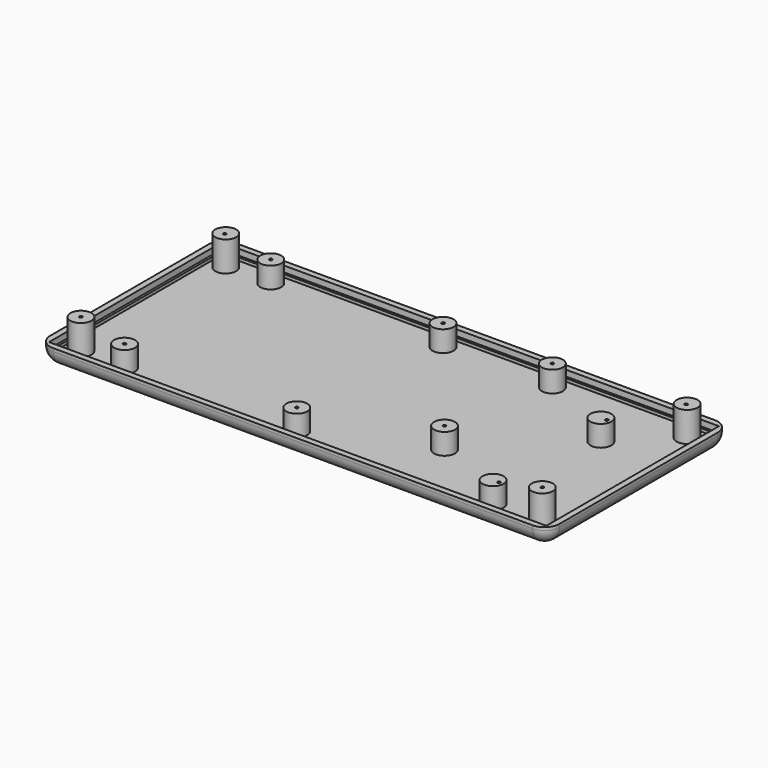
from build123d import *

# Parameters (mm, degrees)
F0_W            = 170
F0_H            = 76
F1_DEPTH        = 6
F2_W            = 164.4
F2_H            = 70.4
F3_DEPTH        = 3
F4_R            = 3.5
F5_DEPTH        = 7
F6_R            = 4
F7_DEPTH        = 2.8
F8_W            = 166
F8_H            = 72
F8_W_2          = 163.2
F8_H_2          = 69.2
F9_DEPTH        = 2
F10_R           = 3.5
F11_DEPTH       = 10
F12_R           = 0.5
F13_DEPTH       = 0.5
F14_R           = 0.5
F15_DEPTH       = 0.5
F17_D           = 3
F17_DEPTH       = 2.5
F17_CSINK_D     = 6.72
F17_CSINK_ANGLE = 90
F17_TIP         = 0.9012909285
F18_T1_DEPTH    = 13.5
F18_T3_DEPTH    = 66
F18_T5_DEPTH    = 160
F18_S9_W        = 5
F18_S9_H        = 5
F18_T10_DEPTH   = 5
F18_S15_W       = 5
F18_S15_H       = 5
F18_T16_DEPTH   = 5
F18_S21_W       = 5
F18_S21_H       = 5
F18_T22_DEPTH   = 5
F18_S27_W       = 5
F18_S27_H       = 5
F18_T28_DEPTH   = 5


# Not quite as in the source:
# - a fillet or chamfer that OpenCascade refuses, or shapes differently, is made with other operations: its cross-section is extruded or revolved along the edge and cut away or added


with BuildPart() as f1:
    # F0 (on Top) → F1 (new body)
    with BuildSketch(Plane.XY):
        with Locations((85, 38)):
            Rectangle(F0_W, F0_H)
    extrude(amount=F1_DEPTH)

    # F2 (on face) → F3 (cut)
    with BuildSketch(Plane.XY.offset(6)):
        with Locations((85, 38)):
            Rectangle(F2_W, F2_H)
    extrude(amount=-F3_DEPTH, mode=Mode.SUBTRACT)

    # F4 (on face) → F5 (join)
    with BuildSketch(Plane.XY.offset(3)):
        with Locations((22.8, 68.5)):
            Circle(F4_R)
        with Locations((22.8, 7.5)):
            Circle(F4_R)
        with Locations((80.3, 68.5)):
            Circle(F4_R)
        with Locations((80.3, 7.5)):
            Circle(F4_R)
        with Locations((116.8, 68.5)):
            Circle(F4_R)
        with Locations((145.8, 52.5)):
            Circle(F4_R)
        with Locations((116.8, 23.5)):
            Circle(F4_R)
        with Locations((145.8, 7.5)):
            Circle(F4_R)
    extrude(amount=F5_DEPTH)

    # F6 (on face) → F7 (cut, through all)
    with BuildSketch(Plane(origin=(0, 0, 0), x_dir=(0, -1, 0), z_dir=(-1, 0, 0))):
        with Locations((-57, 18)):
            Circle(F6_R)
        with Locations((-19, 18)):
            Circle(F6_R)
    extrude(amount=-F7_DEPTH, mode=Mode.SUBTRACT)

    # F8 (on face) → F9 (cut)
    with BuildSketch(Plane.XY.offset(6)):
        with Locations((85, 38)):
            Rectangle(F8_W, F8_H)
        with Locations((84.6, 37.6)):
            Rectangle(F8_W_2, F8_H_2, mode=Mode.SUBTRACT)
    extrude(amount=-F9_DEPTH, mode=Mode.SUBTRACT)

    # F10 (on face) → F11 (join)
    with BuildSketch(Plane.XY.offset(3)):
        with Locations((8, 68.2)):
            Circle(F10_R)
        with Locations((8, 7.8)):
            Circle(F10_R)
        with Locations((162, 7.8)):
            Circle(F10_R)
        with Locations((162, 68.2)):
            Circle(F10_R)
    extrude(amount=F11_DEPTH)

    # F12 (on face) → F13 (cut)
    with BuildSketch(Plane.XY.offset(13)):
        with Locations((8, 67.8)):
            Circle(F12_R)
        with Locations((8, 7.8)):
            Circle(F12_R)
        with Locations((162, 7.8)):
            Circle(F12_R)
        with Locations((162, 67.8)):
            Circle(F12_R)
    extrude(amount=-F13_DEPTH, mode=Mode.SUBTRACT)

    # F14 (on face) → F15 (cut)
    with BuildSketch(Plane.XY.offset(10)):
        with Locations((22.8, 68.5)):
            Circle(F14_R)
        with Locations((22.8, 7.5)):
            Circle(F14_R)
        with Locations((80.3, 68.5)):
            Circle(F14_R)
        with Locations((80.3, 7.5)):
            Circle(F14_R)
        with Locations((116.8, 68.5)):
            Circle(F14_R)
        with Locations((147.8, 52.5)):
            Circle(F14_R)
        with Locations((116.8, 23.5)):
            Circle(F14_R)
        with Locations((147.8, 7.5)):
            Circle(F14_R)
    extrude(amount=-F15_DEPTH, mode=Mode.SUBTRACT)

    # F17
    with Locations(Plane(origin=(0, 0, 0), x_dir=(1, 0, 0), z_dir=(0, 0, -1))):
        with Locations((8, -8), (8, -68), (162, -68), (162, -8)):
            CounterSinkHole(F17_D / 2, F17_CSINK_D / 2, depth=F17_DEPTH, counter_sink_angle=F17_CSINK_ANGLE)
            with Locations((0, 0, -(F17_DEPTH + F17_TIP / 2))):  # 118° drill point
                Cone(0, F17_D / 2, F17_TIP, mode=Mode.SUBTRACT)

    # F18: fillet of radius 5 on 8 edges, made by hand

    # F18_s2 → F18_t1 (cut)
    with BuildSketch(Plane.XY.offset(5)):
        with BuildLine():
            ThreePointArc((165, 76), (168.5355339059, 74.5355339059), (170, 71))
            Line((170, 71), (170, 76))
            Line((170, 76), (165, 76))
        make_face()
        with BuildLine():
            ThreePointArc((165, 0), (168.5355339059, 1.4644660941), (170, 5))
            Line((170, 5), (170, 0))
            Line((170, 0), (165, 0))
        make_face()
        with BuildLine():
            ThreePointArc((0, 71), (1.4644660941, 74.5355339059), (5, 76))
            Line((5, 76), (0, 76))
            Line((0, 76), (0, 71))
        make_face()
        with BuildLine():
            ThreePointArc((0, 5), (1.4644660941, 1.4644660941), (5, 0))
            Line((5, 0), (0, 0))
            Line((0, 0), (0, 5))
        make_face()
    extrude(amount=F18_T1_DEPTH, mode=Mode.SUBTRACT)

    # F18_s4 → F18_t3 (cut)
    with BuildSketch(Plane.XZ.offset(-71)):
        with BuildLine():
            ThreePointArc((165, 0), (168.5355339059, 1.4644660941), (170, 5))
            Line((170, 5), (170, 0))
            Line((170, 0), (165, 0))
        make_face()
        with BuildLine():
            ThreePointArc((0, 5), (1.4644660941, 1.4644660941), (5, 0))
            Line((5, 0), (0, 0))
            Line((0, 0), (0, 5))
        make_face()
    extrude(amount=F18_T3_DEPTH, mode=Mode.SUBTRACT)

    # F18_s6 → F18_t5 (cut)
    with BuildSketch(Plane.YZ.offset(5)):
        with BuildLine():
            ThreePointArc((76, 5), (74.5355339059, 1.4644660941), (71, 0))
            Line((71, 0), (76, 0))
            Line((76, 0), (76, 5))
        make_face()
        with BuildLine():
            ThreePointArc((0, 5), (1.4644660941, 1.4644660941), (5, 0))
            Line((5, 0), (0, 0))
            Line((0, 0), (0, 5))
        make_face()
    extrude(amount=F18_T5_DEPTH, mode=Mode.SUBTRACT)


with BuildPart() as f18_tool8:
    # F18_s9 → F18_t10 (new body)
    with BuildSketch(Plane.XZ.offset(-71)):
        with Locations((167.5, 2.5)):
            Rectangle(F18_S9_W, F18_S9_H)
    extrude(amount=-F18_T10_DEPTH)

    # F18_s11 → F18_t12 (revolve, cut)
    with BuildSketch(Plane(origin=(165, 71, 5), x_dir=(-0.7071067812, 0, 0.7071067812), z_dir=(-0.7071067812, 0, -0.7071067812))):
        with BuildLine():
            ThreePointArc((0, -5), (5, 0), (0, 5))
            Line((0, 5), (0, -5))
        make_face()
    revolve(axis=Axis((165, 71, 5), (0, 1, 0)), mode=Mode.SUBTRACT)


with BuildPart() as f1_1:
    add(f1.part)

    # F18_t7: cut F18_tool8
    add(f18_tool8.part, mode=Mode.SUBTRACT)


with BuildPart() as f18_tool14:
    # F18_s15 → F18_t16 (new body)
    with BuildSketch(Plane.XZ.offset(-5)):
        with Locations((167.5, 2.5)):
            Rectangle(F18_S15_W, F18_S15_H)
    extrude(amount=F18_T16_DEPTH)

    # F18_s17 → F18_t18 (revolve, cut)
    with BuildSketch(Plane(origin=(165, 5, 5), x_dir=(-0.7071067812, 0, 0.7071067812), z_dir=(0.7071067812, 0, 0.7071067812))):
        with BuildLine():
            ThreePointArc((0, -5), (5, 0), (0, 5))
            Line((0, 5), (0, -5))
        make_face()
    revolve(axis=Axis((165, 5, 5), (0, -1, 0)), mode=Mode.SUBTRACT)


with BuildPart() as f1_2:
    add(f1_1.part)

    # F18_t13: cut F18_tool14
    add(f18_tool14.part, mode=Mode.SUBTRACT)


with BuildPart() as f18_tool20:
    # F18_s21 → F18_t22 (new body)
    with BuildSketch(Plane.YZ.offset(5)):
        with Locations((73.5, 2.5)):
            Rectangle(F18_S21_W, F18_S21_H)
    extrude(amount=-F18_T22_DEPTH)

    # F18_s23 → F18_t24 (revolve, cut)
    with BuildSketch(Plane(origin=(5, 71, 5), x_dir=(0, -0.7071067812, 0.7071067812), z_dir=(0, -0.7071067812, -0.7071067812))):
        with BuildLine():
            ThreePointArc((0, -5), (5, 0), (0, 5))
            Line((0, 5), (0, -5))
        make_face()
    revolve(axis=Axis((5, 71, 5), (-1, 0, 0)), mode=Mode.SUBTRACT)


with BuildPart() as f1_3:
    add(f1_2.part)

    # F18_t19: cut F18_tool20
    add(f18_tool20.part, mode=Mode.SUBTRACT)


with BuildPart() as f18_tool26:
    # F18_s27 → F18_t28 (new body)
    with BuildSketch(Plane.YZ.offset(5)):
        with Locations((2.5, 2.5)):
            Rectangle(F18_S27_W, F18_S27_H)
    extrude(amount=-F18_T28_DEPTH)

    # F18_s29 → F18_t30 (revolve, cut)
    with BuildSketch(Plane(origin=(5, 5, 5), x_dir=(0, 0.7071067812, 0.7071067812), z_dir=(0, -0.7071067812, 0.7071067812))):
        with BuildLine():
            ThreePointArc((0, -5), (5, 0), (0, 5))
            Line((0, 5), (0, -5))
        make_face()
    revolve(axis=Axis((5, 5, 5), (-1, 0, 0)), mode=Mode.SUBTRACT)


with BuildPart() as f1_4:
    add(f1_3.part)

    # F18_t25: cut F18_tool26
    add(f18_tool26.part, mode=Mode.SUBTRACT)


solid = f1_4.part
